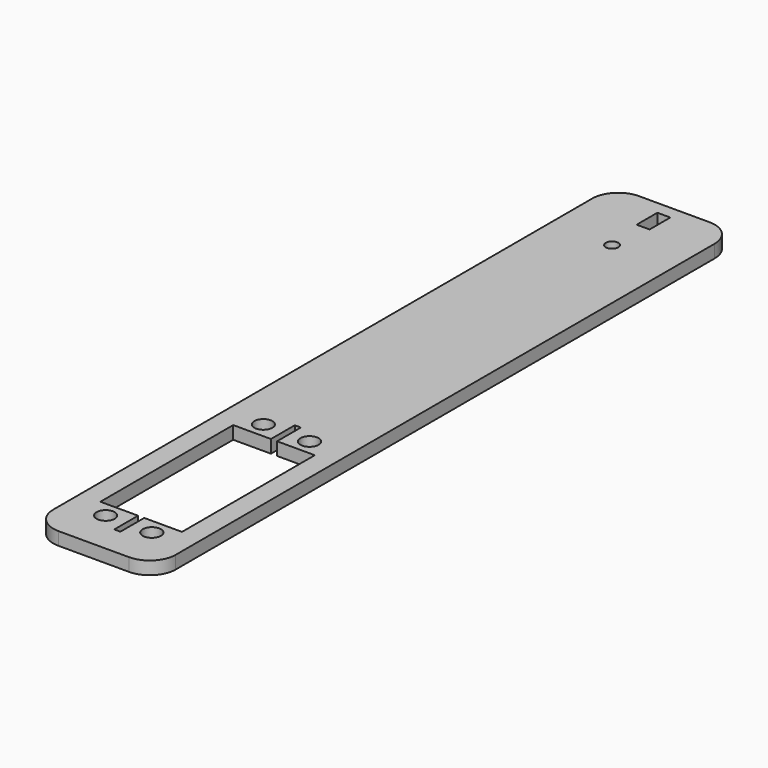
from build123d import *

# Parameters (mm, degrees)
F0_R     = 2.2225
F0_R_2   = 1.524
F0_W     = 3.175
F0_H     = 6.35
F1_DEPTH = 3.175


# Not quite as in the source:
# - a length typed as a fraction of an inch, garbled in the dataset ("3 / 203.2 mm" for 3/8 in), is restored


with BuildPart() as f1:
    # F0 (on Top) → F1 (new body)
    with BuildSketch(Plane.XY):
        with BuildLine():
            ThreePointArc((15, 82.55), (13.1401280605, 87.0401280605), (8.65, 88.9))
            Line((8.65, 88.9), (-8.65, 88.9))
            ThreePointArc((-8.65, 88.9), (-13.1401280605, 87.0401280605), (-15, 82.55))
            Line((-15, 82.55), (-15, -82.55))
            ThreePointArc((-15, -82.55), (-13.1401280605, -87.0401280605), (-8.65, -88.9))
            Line((-8.65, -88.9), (8.65, -88.9))
            ThreePointArc((8.65, -88.9), (13.1401280605, -87.0401280605), (15, -82.55))
            Line((15, -82.55), (15, 82.55))
        make_face()
        with Locations((-5.6566, -78.197214059)):
            Circle(F0_R, mode=Mode.SUBTRACT)
        Polygon((0.75, -33.696414059), (10, -33.696414059), (10, -74.387214059), (0.75, -74.387214059), (0.75, -81.691814059), (-0.75, -81.691814059), (-0.75, -74.387214059), (-10, -74.387214059), (-10, -33.696414059), (-0.75, -33.696414059), (-0.75, -26.391814059), (0.75, -26.391814059), align=None, mode=Mode.SUBTRACT)
        with Locations((-5.6566, -29.886414059)):
            Circle(F0_R, mode=Mode.SUBTRACT)
        with Locations((5.6566, -78.197214059)):
            Circle(F0_R, mode=Mode.SUBTRACT)
        with Locations((5.6566, -29.886414059)):
            Circle(F0_R, mode=Mode.SUBTRACT)
        with Locations((0, 69.85)):
            Circle(F0_R_2, mode=Mode.SUBTRACT)
        with Locations((0, 82.55)):
            Rectangle(F0_W, F0_H, mode=Mode.SUBTRACT)
    extrude(amount=F1_DEPTH)


solid = f1.part
